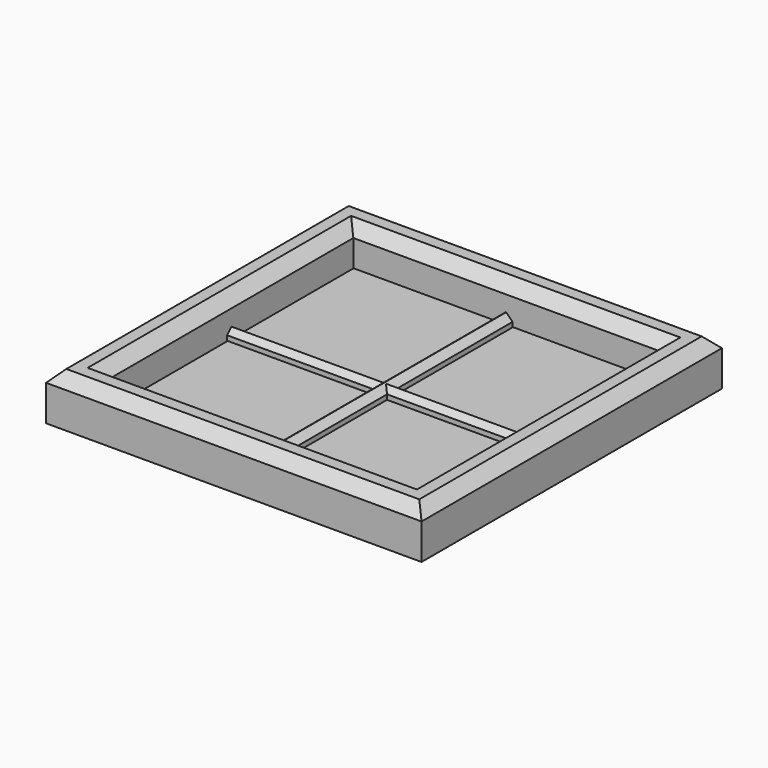
from build123d import *

# Parameters (mm, degrees)
F0_W         = 25.4
F0_H         = 25.4
F0_W_2       = 20.7499843091
F0_H_2       = 20.7499843091
F1_DEPTH     = 3.175
F2_W         = 20.6769648939
F2_H         = 20.6769648939
F3_DEPTH     = 0.635
F5_W         = 0.8874461055
F5_H         = 9.8797418177
F5_H_2       = 0.7302556187
F5_W_2       = 10.0232437253
F5_W_3       = 10.0361239165
F5_H_3       = 10.0780427456
F6_DEPTH     = 0.762
F7_T1_DEPTH  = 11.1336964395
F7_T3_DEPTH  = 10.9901945319
F7_T5_DEPTH  = 11.1465766307
F7_T7_DEPTH  = 11.1884954598
F7_T12_DEPTH = 12.2441491537
F7_T17_DEPTH = 12.2441491537
F7_T22_DEPTH = 12.1006472461
F7_T27_DEPTH = 12.1006472461
F7_T32_DEPTH = 12.2570293449
F7_T37_DEPTH = 12.2570293449
F7_T42_DEPTH = 12.298948174
F7_T47_DEPTH = 12.298948174
F7_T53_DEPTH = 12.2441491537
F7_T58_DEPTH = 12.298948174
F7_T66_DEPTH = 12.1006472461
F7_T71_DEPTH = 12.2441491537
F7_T79_DEPTH = 12.2570293449
F7_T84_DEPTH = 12.1006472461
F7_T92_DEPTH = 12.298948174
F7_T97_DEPTH = 12.2570293449
F8_SIZE      = 0.762


# Not quite as in the source:
# - a fillet or chamfer that OpenCascade refuses, or shapes differently, is made with other operations: its cross-section is extruded or revolved along the edge and cut away or added


with BuildPart() as f1:
    # F0 (on Top) → F1 (new body)
    with BuildSketch(Plane.XY):
        with Locations((-27.3323692381, -29.8893228173)):
            Rectangle(F0_W, F0_H)
        with Locations((-27.3323692381, -29.8893228173)):
            Rectangle(F0_W_2, F0_H_2, mode=Mode.SUBTRACT)
    extrude(amount=F1_DEPTH)

    # F8
    f8_edges = [f1.edges().sort_by_distance(p)[0] for p in [
        (-14.632369, -29.889323, 3.175),
        (-27.332369, -42.589323, 3.175),
        (-40.032369, -29.889323, 3.175),
        (-27.332369, -17.189323, 3.175),
        (-37.707361, -29.889323, 3.175),
        (-27.332369, -19.514331, 3.175),
        (-16.957377, -29.889323, 3.175),
        (-27.332369, -40.264315, 3.175),
    ]]
    chamfer(f8_edges, length=F8_SIZE)


with BuildPart() as f3:
    # F2 (on Top) → F3 (new body)
    with BuildSketch(Plane.XY):
        with Locations((-27.32637804, -29.8832794651)):
            Rectangle(F2_W, F2_H)
    extrude(amount=F3_DEPTH)


with BuildPart() as f6:
    # F5 (on face) → F6 (new body)
    with BuildSketch(Plane.XY.offset(0.635)):
        with Locations((-27.3266136646, -24.5234593749)):
            Rectangle(F5_W, F5_H)
        with Locations((-27.3266136646, -29.8284580931)):
            Rectangle(F5_W, F5_H_2)
        with Locations((-32.78195858, -29.8284580931)):
            Rectangle(F5_W_2, F5_H_2)
        with Locations((-21.8648286536, -29.8284580931)):
            Rectangle(F5_W_3, F5_H_2)
        with Locations((-27.3266136646, -35.2326072752)):
            Rectangle(F5_W, F5_H_3)
    extrude(amount=F6_DEPTH)

    # F7: chamfer of 0.4318 on 8 edges, made by hand

    # F7_s2 → F7_t1 (cut)
    with BuildSketch(Plane.YZ.offset(-38.9040331569)):
        Polygon((-30.1935859025, 0.9652), (-29.7617859025, 1.397), (-30.1935859025, 1.397), align=None)
        Polygon((-29.4633302838, 0.9652), (-29.8951302838, 1.397), (-29.4633302838, 1.397), align=None)
    extrude(amount=F7_T1_DEPTH, mode=Mode.SUBTRACT)

    # F7_s4 → F7_t3 (cut)
    with BuildSketch(Plane.XZ.offset(18.4731357518)):
        Polygon((-27.7703367174, 0.9652), (-27.3385367174, 1.397), (-27.7703367174, 1.397), align=None)
        Polygon((-26.8828906119, 0.9652), (-27.3146906119, 1.397), (-26.8828906119, 1.397), align=None)
    extrude(amount=F7_T3_DEPTH, mode=Mode.SUBTRACT)

    # F7_s6 → F7_t5 (cut)
    with BuildSketch(Plane.YZ.offset(-26.8828906119)):
        Polygon((-29.4633302838, 0.9652), (-29.8951302838, 1.397), (-29.4633302838, 1.397), align=None)
        Polygon((-30.1935859025, 0.9652), (-29.7617859025, 1.397), (-30.1935859025, 1.397), align=None)
    extrude(amount=F7_T5_DEPTH, mode=Mode.SUBTRACT)

    # F7_s8 → F7_t7 (cut)
    with BuildSketch(Plane.XZ.offset(30.1935859025)):
        Polygon((-26.8828906119, 0.9652), (-27.3146906119, 1.397), (-26.8828906119, 1.397), align=None)
        Polygon((-27.7703367174, 0.9652), (-27.3385367174, 1.397), (-27.7703367174, 1.397), align=None)
    extrude(amount=F7_T7_DEPTH, mode=Mode.SUBTRACT)


with BuildPart() as f7_tool10:
    # F7_s11 → F7_t12 (new body)
    with BuildSketch(Plane.YZ.offset(-38.9040331569)):
        Polygon((-30.1935859025, 0.9652), (-29.7617859025, 1.397), (-30.1935859025, 1.397), align=None)
    extrude(amount=F7_T12_DEPTH)

    split(bisect_by=Plane.YZ.offset(-26.8828906119), keep=Keep.TOP)


with BuildPart() as f6_1:
    add(f6.part)

    # F7_t9: cut F7_tool10
    add(f7_tool10.part, mode=Mode.SUBTRACT)


with BuildPart() as f7_tool15:
    # F7_s16 → F7_t17 (new body)
    with BuildSketch(Plane.YZ.offset(-26.6598840032)):
        Polygon((-29.4633302838, 0.9652), (-29.8951302838, 1.397), (-29.4633302838, 1.397), align=None)
    extrude(amount=-F7_T17_DEPTH)

    split(bisect_by=Plane.YZ.offset(-26.8828906119), keep=Keep.TOP)


with BuildPart() as f6_2:
    add(f6_1.part)

    # F7_t14: cut F7_tool15
    add(f7_tool15.part, mode=Mode.SUBTRACT)


with BuildPart() as f7_tool20:
    # F7_s21 → F7_t22 (new body)
    with BuildSketch(Plane.XZ.offset(18.4731357518)):
        Polygon((-27.7703367174, 0.9652), (-27.3385367174, 1.397), (-27.7703367174, 1.397), align=None)
    extrude(amount=F7_T22_DEPTH)

    split(bisect_by=Plane.XZ.offset(30.1935859025), keep=Keep.TOP)


with BuildPart() as f6_3:
    add(f6_2.part)

    # F7_t19: cut F7_tool20
    add(f7_tool20.part, mode=Mode.SUBTRACT)


with BuildPart() as f7_tool25:
    # F7_s26 → F7_t27 (new body)
    with BuildSketch(Plane.XZ.offset(30.573782998)):
        Polygon((-26.8828906119, 0.9652), (-27.3146906119, 1.397), (-26.8828906119, 1.397), align=None)
    extrude(amount=-F7_T27_DEPTH)

    split(bisect_by=Plane.XZ.offset(30.1935859025), keep=Keep.TOP)


with BuildPart() as f6_4:
    add(f6_3.part)

    # F7_t24: cut F7_tool25
    add(f7_tool25.part, mode=Mode.SUBTRACT)


with BuildPart() as f7_tool30:
    # F7_s31 → F7_t32 (new body)
    with BuildSketch(Plane.YZ.offset(-15.7363139812)):
        Polygon((-29.4633302838, 0.9652), (-29.8951302838, 1.397), (-29.4633302838, 1.397), align=None)
    extrude(amount=-F7_T32_DEPTH)

    split(bisect_by=Plane.YZ.offset(-27.7703367174), keep=Keep.BOTTOM)


with BuildPart() as f6_5:
    add(f6_4.part)

    # F7_t29: cut F7_tool30
    add(f7_tool30.part, mode=Mode.SUBTRACT)


with BuildPart() as f7_tool35:
    # F7_s36 → F7_t37 (new body)
    with BuildSketch(Plane.YZ.offset(-27.9933433261)):
        Polygon((-30.1935859025, 0.9652), (-29.7617859025, 1.397), (-30.1935859025, 1.397), align=None)
    extrude(amount=F7_T37_DEPTH)

    split(bisect_by=Plane.YZ.offset(-27.7703367174), keep=Keep.BOTTOM)


with BuildPart() as f6_6:
    add(f6_5.part)

    # F7_t34: cut F7_tool35
    add(f7_tool35.part, mode=Mode.SUBTRACT)


with BuildPart() as f7_tool40:
    # F7_s41 → F7_t42 (new body)
    with BuildSketch(Plane.XZ.offset(41.3820813622)):
        Polygon((-26.8828906119, 0.9652), (-27.3146906119, 1.397), (-26.8828906119, 1.397), align=None)
    extrude(amount=-F7_T42_DEPTH)

    split(bisect_by=Plane.XZ.offset(29.4633302838), keep=Keep.BOTTOM)


with BuildPart() as f6_7:
    add(f6_6.part)

    # F7_t39: cut F7_tool40
    add(f7_tool40.part, mode=Mode.SUBTRACT)


with BuildPart() as f7_tool45:
    # F7_s46 → F7_t47 (new body)
    with BuildSketch(Plane.XZ.offset(29.0831331882)):
        Polygon((-27.7703367174, 0.9652), (-27.3385367174, 1.397), (-27.7703367174, 1.397), align=None)
    extrude(amount=F7_T47_DEPTH)

    split(bisect_by=Plane.XZ.offset(29.4633302838), keep=Keep.BOTTOM)


with BuildPart() as f6_8:
    add(f6_7.part)

    # F7_t44: cut F7_tool45
    add(f7_tool45.part, mode=Mode.SUBTRACT)


with BuildPart() as f7_tool51:
    # F7_s52 → F7_t53 (new body)
    with BuildSketch(Plane.YZ.offset(-38.9040331569)):
        Polygon((-30.1935859025, 0.9652), (-29.7617859025, 1.397), (-30.1935859025, 1.397), align=None)
    extrude(amount=F7_T53_DEPTH)

    split(bisect_by=Plane.YZ.offset(-27.7703367174), keep=Keep.TOP)

    split(bisect_by=Plane.YZ.offset(-26.8828906119), keep=Keep.BOTTOM)


with BuildPart() as f7_tool56:
    # F7_s57 → F7_t58 (new body)
    with BuildSketch(Plane.XZ.offset(29.0831331882)):
        Polygon((-27.7703367174, 0.9652), (-27.3385367174, 1.397), (-27.7703367174, 1.397), align=None)
    extrude(amount=F7_T58_DEPTH)

    split(bisect_by=Plane.XZ.offset(29.4633302838), keep=Keep.TOP)

    split(bisect_by=Plane.XZ.offset(30.1935859025), keep=Keep.BOTTOM)


with BuildPart() as f7_tool51_1:
    add(f7_tool51.part)

    # F7_t61: intersect F7_tool56
    add(f7_tool56.part, mode=Mode.INTERSECT)


with BuildPart() as f6_9:
    add(f6_8.part)

    # F7_t49: cut F7_tool51
    add(f7_tool51_1.part, mode=Mode.SUBTRACT)


with BuildPart() as f7_tool64:
    # F7_s65 → F7_t66 (new body)
    with BuildSketch(Plane.XZ.offset(18.4731357518)):
        Polygon((-27.7703367174, 0.9652), (-27.3385367174, 1.397), (-27.7703367174, 1.397), align=None)
    extrude(amount=F7_T66_DEPTH)

    split(bisect_by=Plane.XZ.offset(29.4633302838), keep=Keep.TOP)

    split(bisect_by=Plane.XZ.offset(30.1935859025), keep=Keep.BOTTOM)


with BuildPart() as f7_tool69:
    # F7_s70 → F7_t71 (new body)
    with BuildSketch(Plane.YZ.offset(-26.6598840032)):
        Polygon((-29.4633302838, 0.9652), (-29.8951302838, 1.397), (-29.4633302838, 1.397), align=None)
    extrude(amount=-F7_T71_DEPTH)

    split(bisect_by=Plane.YZ.offset(-27.7703367174), keep=Keep.TOP)

    split(bisect_by=Plane.YZ.offset(-26.8828906119), keep=Keep.BOTTOM)


with BuildPart() as f7_tool64_1:
    add(f7_tool64.part)

    # F7_t74: intersect F7_tool69
    add(f7_tool69.part, mode=Mode.INTERSECT)


with BuildPart() as f6_10:
    add(f6_9.part)

    # F7_t62: cut F7_tool64
    add(f7_tool64_1.part, mode=Mode.SUBTRACT)


with BuildPart() as f7_tool77:
    # F7_s78 → F7_t79 (new body)
    with BuildSketch(Plane.YZ.offset(-15.7363139812)):
        Polygon((-29.4633302838, 0.9652), (-29.8951302838, 1.397), (-29.4633302838, 1.397), align=None)
    extrude(amount=-F7_T79_DEPTH)

    split(bisect_by=Plane.YZ.offset(-27.7703367174), keep=Keep.TOP)

    split(bisect_by=Plane.YZ.offset(-26.8828906119), keep=Keep.BOTTOM)


with BuildPart() as f7_tool82:
    # F7_s83 → F7_t84 (new body)
    with BuildSketch(Plane.XZ.offset(30.573782998)):
        Polygon((-26.8828906119, 0.9652), (-27.3146906119, 1.397), (-26.8828906119, 1.397), align=None)
    extrude(amount=-F7_T84_DEPTH)

    split(bisect_by=Plane.XZ.offset(30.1935859025), keep=Keep.BOTTOM)

    split(bisect_by=Plane.XZ.offset(29.4633302838), keep=Keep.TOP)


with BuildPart() as f7_tool77_1:
    add(f7_tool77.part)

    # F7_t87: intersect F7_tool82
    add(f7_tool82.part, mode=Mode.INTERSECT)


with BuildPart() as f6_11:
    add(f6_10.part)

    # F7_t75: cut F7_tool77
    add(f7_tool77_1.part, mode=Mode.SUBTRACT)


with BuildPart() as f7_tool90:
    # F7_s91 → F7_t92 (new body)
    with BuildSketch(Plane.XZ.offset(41.3820813622)):
        Polygon((-26.8828906119, 0.9652), (-27.3146906119, 1.397), (-26.8828906119, 1.397), align=None)
    extrude(amount=-F7_T92_DEPTH)

    split(bisect_by=Plane.XZ.offset(30.1935859025), keep=Keep.BOTTOM)

    split(bisect_by=Plane.XZ.offset(29.4633302838), keep=Keep.TOP)


with BuildPart() as f7_tool95:
    # F7_s96 → F7_t97 (new body)
    with BuildSketch(Plane.YZ.offset(-27.9933433261)):
        Polygon((-30.1935859025, 0.9652), (-29.7617859025, 1.397), (-30.1935859025, 1.397), align=None)
    extrude(amount=F7_T97_DEPTH)

    split(bisect_by=Plane.YZ.offset(-27.7703367174), keep=Keep.TOP)

    split(bisect_by=Plane.YZ.offset(-26.8828906119), keep=Keep.BOTTOM)


with BuildPart() as f7_tool90_1:
    add(f7_tool90.part)

    # F7_t100: intersect F7_tool95
    add(f7_tool95.part, mode=Mode.INTERSECT)


with BuildPart() as f6_12:
    add(f6_11.part)

    # F7_t88: cut F7_tool90
    add(f7_tool90_1.part, mode=Mode.SUBTRACT)


solid = Compound([f1.part, f3.part, f6_12.part])
